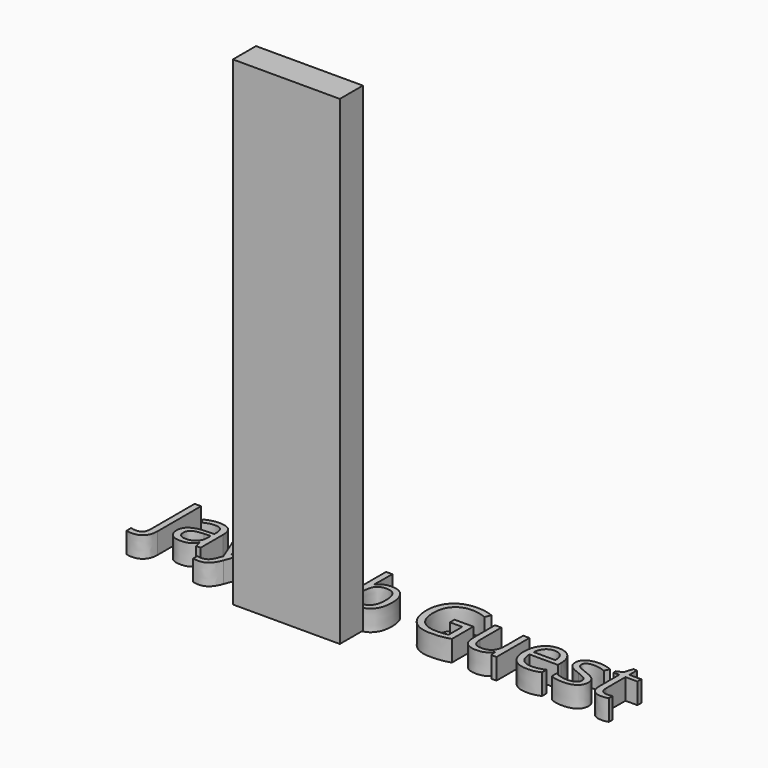
from build123d import *

# Parameters (mm, degrees)
F0_TEXT_SIZE = 93.7352060444
F1_DEPTH     = 25.4
F2_R         = 12.9117500037
F2_R_2       = 10.4577209846
F2_R_3       = 8.407521812
F4_DEPTH     = 25.4
F2_R_4       = 3.2664432934
F6_W         = 130.150437355
F6_H         = 35.1199582219
F7_DEPTH     = 584.2


# Not quite as in the source:
# - Text() gives the source's letters only with a copy of the font that has no kerning and outlines rounded to 1/6400 em; it was checked with that copy


with BuildPart() as f1:
    # F0 (on Top) → F1 (new body)
    with BuildSketch(Plane.XY):
        with Locations((-83.9799642563, -18.3228999376)):
            Text('Jaykob Guest', F0_TEXT_SIZE, font='Open Sans', text_align=(TextAlign.LEFT, TextAlign.BOTTOM))
    extrude(amount=F1_DEPTH)


with BuildPart() as f4:
    # F2 (on face) → F4 (new body)
    with BuildSketch(Plane.XY.offset(25.4)):
        with Locations((117.4738258123, 4.9933446571)):
            Circle(F2_R)
        with Locations((117.4738258123, 4.9933446571)):
            Circle(F2_R_2, mode=Mode.SUBTRACT)
        with Locations((117.4738258123, 4.9933446571)):
            Circle(F2_R_2)
        with Locations((117.4738258123, 4.9933446571)):
            Circle(F2_R_3, mode=Mode.SUBTRACT)
    extrude(amount=F4_DEPTH)


with BuildPart() as f4b:
    # F2 (on face) → F4, piece 2 (new body)
    with BuildSketch(Plane.XY.offset(25.4)):
        with Locations((117.4738258123, 4.9933446571)):
            Circle(F2_R_4)
    extrude(amount=F4_DEPTH)


with BuildPart() as f7:
    # F6 (on face) → F7 (new body)
    with BuildSketch(Plane.XY.offset(25.4)):
        with Locations((147.6873159409, -72.965465486)):
            Rectangle(F6_W, F6_H)
    extrude(amount=F7_DEPTH)


solid = Compound([f1.part, f4.part, f4b.part, f7.part])
